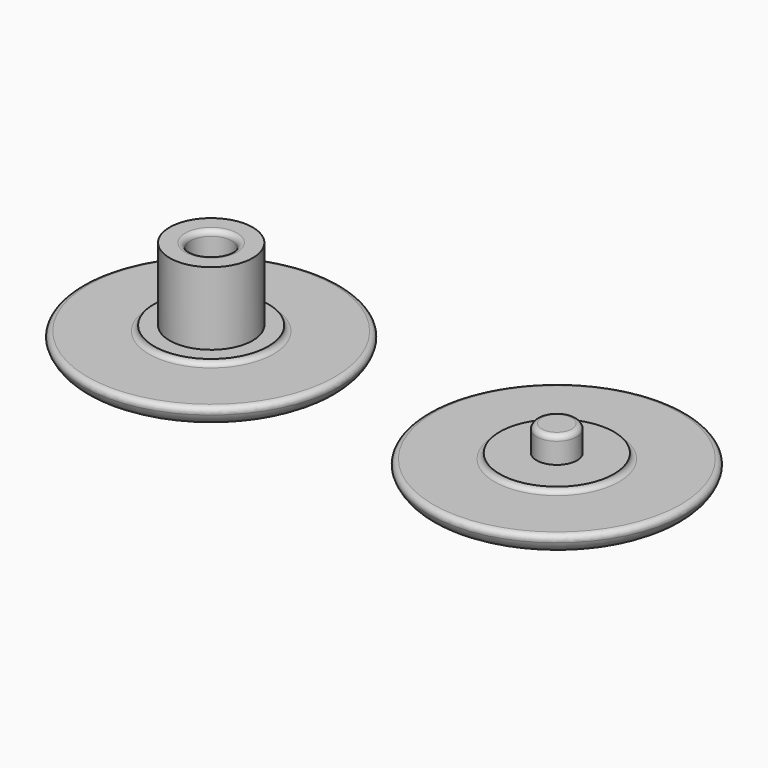
from build123d import *

# Parameters (mm, degrees)
F0_R     = 12.5
F0_R_2   = 5.5
F1_DEPTH = 2
F0_R_3   = 4
F2_DEPTH = 2.5
F0_R_4   = 1.95
F0_R_5   = 2
F3_DEPTH = 9.5
F4_DEPTH = 5
F7_R     = 1.99999
F8_R     = 0.49999


# Not quite as in the source:
# - a fillet or chamfer is up to 0.001 mm smaller than in the source, because OpenCascade refuses the exact size


with BuildPart() as f1:
    # F0 (on Top) → F1 (new body)
    with BuildSketch(Plane.XY):
        with Locations((-165.7585352659, 137.4950408936)):
            Circle(F0_R)
        with Locations((-165.7585352659, 137.4950408936)):
            Circle(F0_R_2, mode=Mode.SUBTRACT)
    extrude(amount=F1_DEPTH)


with BuildPart() as f1b:
    # F0 (on Top) → F1, piece 2 (new body)
    with BuildSketch(Plane.XY):
        with Locations((-132.4781477451, 137.4950408936)):
            Circle(F0_R)
        with Locations((-132.4781477451, 137.4950408936)):
            Circle(F0_R_2, mode=Mode.SUBTRACT)
    extrude(amount=F1_DEPTH)


with BuildPart() as f2:
    # F0 (on Top) → F2 (new body)
    with BuildSketch(Plane.XY):
        with Locations((-165.7585352659, 137.4950408936)):
            Circle(F0_R_2)
        with Locations((-165.7585352659, 137.4950408936)):
            Circle(F0_R_3, mode=Mode.SUBTRACT)
    extrude(amount=F2_DEPTH)


with BuildPart() as f2b:
    # F0 (on Top) → F2, piece 2 (new body)
    with BuildSketch(Plane.XY):
        with Locations((-132.4781477451, 137.4950408936)):
            Circle(F0_R_2)
        with Locations((-132.4781477451, 137.4950408936)):
            Circle(F0_R_4, mode=Mode.SUBTRACT)
    extrude(amount=F2_DEPTH)

    # F0 (on Top) → F4 (join)
    with BuildSketch(Plane.XY):
        with Locations((-132.4781477451, 137.4950408936)):
            Circle(F0_R_4)
    extrude(amount=F4_DEPTH)


with BuildPart() as f2c:
    # F0 (on Top) → F2, piece 3 (new body)
    with BuildSketch(Plane.XY):
        with Locations((-165.7585352659, 137.4950408936)):
            Circle(F0_R_5)
    extrude(amount=F2_DEPTH)


with BuildPart() as f3:
    # F0 (on Top) → F3 (new body)
    with BuildSketch(Plane.XY):
        with Locations((-165.7585352659, 137.4950408936)):
            Circle(F0_R_3)
        with Locations((-165.7585352659, 137.4950408936)):
            Circle(F0_R_5, mode=Mode.SUBTRACT)
    extrude(amount=F3_DEPTH)

    # F5: union F2c, F1, F2
    add(f2c.part)
    add(f1.part)
    add(f2.part)

    # F6: union F2b, F1b
    add(f2b.part)
    add(f1b.part)

    # F7 (radius 2 in the source; OpenCascade refuses exactly that, so slightly less here)
    f7_edges = [f3.edges().sort_by_distance(p)[0] for p in [
        (-144.978148, 137.495041, 0),
        (-178.258535, 137.495041, 0),
    ]]
    fillet(f7_edges, radius=F7_R)

    # F8 (radius 0.5 in the source; OpenCascade refuses exactly that, so slightly less here)
    f8_edges = [f3.edges().sort_by_distance(p)[0] for p in [
        (-178.258535, 137.495041, 2),
        (-171.258535, 137.495041, 2),
        (-144.978148, 137.495041, 2),
        (-137.978148, 137.495041, 2),
        (-134.428148, 137.495041, 5),
        (-167.758535, 137.495041, 9.5),
    ]]
    fillet(f8_edges, radius=F8_R)


solid = f3.part
